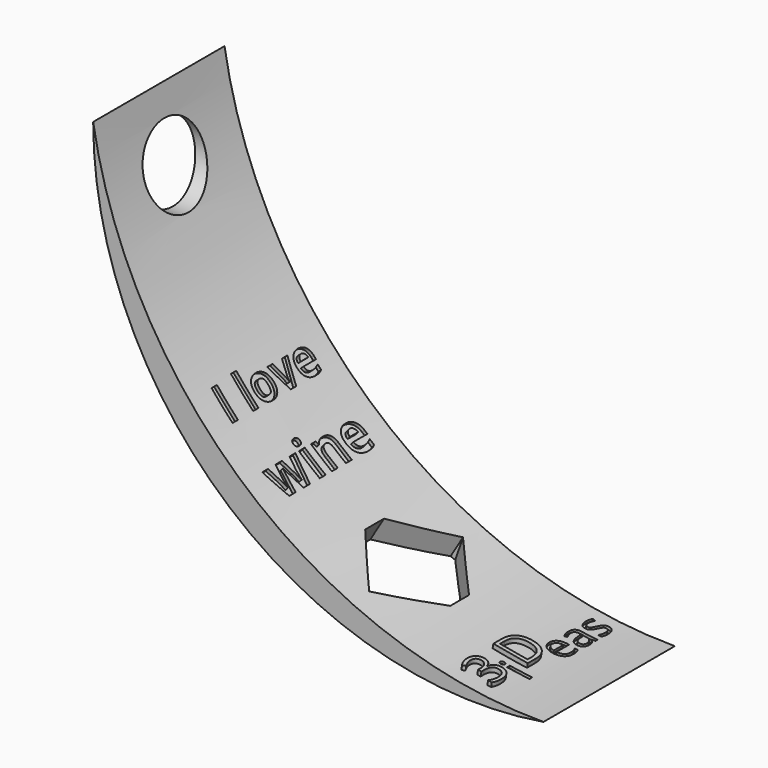
from build123d import *

# Parameters (mm, degrees)
F1_DEPTH      = 70
F3_TEXT_SIZE  = 18.9967349362
F4_DEPTH      = 1.5
F5_R          = 16
F6_DEPTH      = 25
F8_TEXT_SIZE  = 21.1318761144
F9_DEPTH      = 1.5
F11_TEXT_SIZE = 20.8333333333
F12_DEPTH     = 2
F13_TEXT_SIZE = 18.0555555556
F14_DEPTH     = 1
F17_DEPTH     = 25
F18_SIZE      = 19.999


# Not quite as in the source:
# - a fillet or chamfer is up to 0.001 mm smaller than in the source, because OpenCascade refuses the exact size
# - Text() gives the source's letters only with a copy of the font that has no kerning and outlines rounded to 1/6400 em; it was checked with that copy


with BuildPart() as f1:
    # F0 (on Front) → F1 (new body)
    with BuildSketch(Plane.XZ):
        with BuildLine():
            ThreePointArc((192, 0), (66.0595220255, 46.0720986713), (0, 162.775919595))
            ThreePointArc((0, 162.775919595), (58.2994845373, 36.9188578146), (192, 0))
        make_face()
    extrude(amount=F1_DEPTH)

    # F3 (on face) → F4 (cut, symmetric)
    with BuildSketch(Plane(origin=(58.6403576125, 0, 51.2872980146), x_dir=(0, 1, 0), z_dir=(0.7527230816, 0, 0.6583372711))):
        with Locations((-60, 13.1774220479)):
            Text('I love', F3_TEXT_SIZE, font='Open Sans', font_style=FontStyle.BOLD, text_align=(TextAlign.LEFT, TextAlign.BOTTOM))
    extrude(amount=F4_DEPTH, both=True, mode=Mode.SUBTRACT)

    # F5 (on Right) → F6 (cut)
    with BuildSketch(Plane.YZ):
        with Locations((-35, 134.775919595)):
            Circle(F5_R)
    extrude(amount=F6_DEPTH, mode=Mode.SUBTRACT)

    # F8 (on face) → F9 (cut, symmetric)
    with BuildSketch(Plane(origin=(49.9367113152, 0, 59.5810753597), x_dir=(0.7664100857, 0, -0.6423516019), z_dir=(0.6423516019, 0, 0.7664100857))):
        with Locations(Location((29.7385072129, -60), (0, 0, 90))):
            Text('wine', F8_TEXT_SIZE, font='Open Sans', font_style=FontStyle.BOLD, text_align=(TextAlign.LEFT, TextAlign.BOTTOM))
    extrude(amount=F9_DEPTH, both=True, mode=Mode.SUBTRACT)

    # F11 (on line) → F12 (join)
    with BuildSketch(Plane(origin=(5.2267098671, 0, 29.7643801742), x_dir=(0.9849294782, 0, -0.1729564194), z_dir=(0.1729564194, 0, 0.9849294782))):
        with Locations(Location((162.671178636, -65), (0, 0, 90))):
            Text('3 D', F11_TEXT_SIZE, font='Open Sans', text_align=(TextAlign.LEFT, TextAlign.BOTTOM))
    extrude(amount=F12_DEPTH)

    # F13 (on line) → F14 (cut, symmetric)
    with BuildSketch(Plane(origin=(5.2267098671, 0, 29.7643801742), x_dir=(0.9849294782, 0, -0.1729564194), z_dir=(0.1729564194, 0, 0.9849294782))):
        with Locations(Location((167.671178636, -52), (0, 0, 90))):
            Text('i', F13_TEXT_SIZE, font='Open Sans', text_align=(TextAlign.LEFT, TextAlign.BOTTOM))
        with Locations(Location((167.671178636, -32.955078125), (0, 0, 90))):
            Text('eas', F13_TEXT_SIZE, font='Open Sans', text_align=(TextAlign.LEFT, TextAlign.BOTTOM))
    extrude(amount=F14_DEPTH, both=True, mode=Mode.SUBTRACT)

    # F16 (on face) → F17 (cut, symmetric)
    with BuildSketch(Plane(origin=(0, -35, 0), x_dir=(-1, 0, 0), z_dir=(0, 1, 0))):
        with BuildLine():
            ThreePointArc((-91.9887288654, 27.5204363667), (-109.6844712328, 18.1435030463), (-128.2517795117, 10.6387552354))
            Line((-128.2517795117, 10.6387552354), (-125.4690919569, 2.5813275849))
            ThreePointArc((-125.4690919569, 2.5813275849), (-105.3395295061, 8.9395511367), (-86.1865060525, 17.8158106968))
            Line((-86.1865060525, 17.8158106968), (-91.9887288654, 27.5204363667))
        make_face()
    extrude(amount=F17_DEPTH, both=True, mode=Mode.SUBTRACT)

    # F18 (size 20 in the source; OpenCascade refuses exactly that, so slightly less here)
    f18_edges = [f1.edges().sort_by_distance(p)[0] for p in [
        (89.087617, -10, 22.668124),
        (89.087617, -60, 22.668124),
        (126.860436, -60, 6.610041),
        (126.860436, -10, 6.610041),
    ]]
    chamfer(f18_edges, length=F18_SIZE)


solid = f1.part
